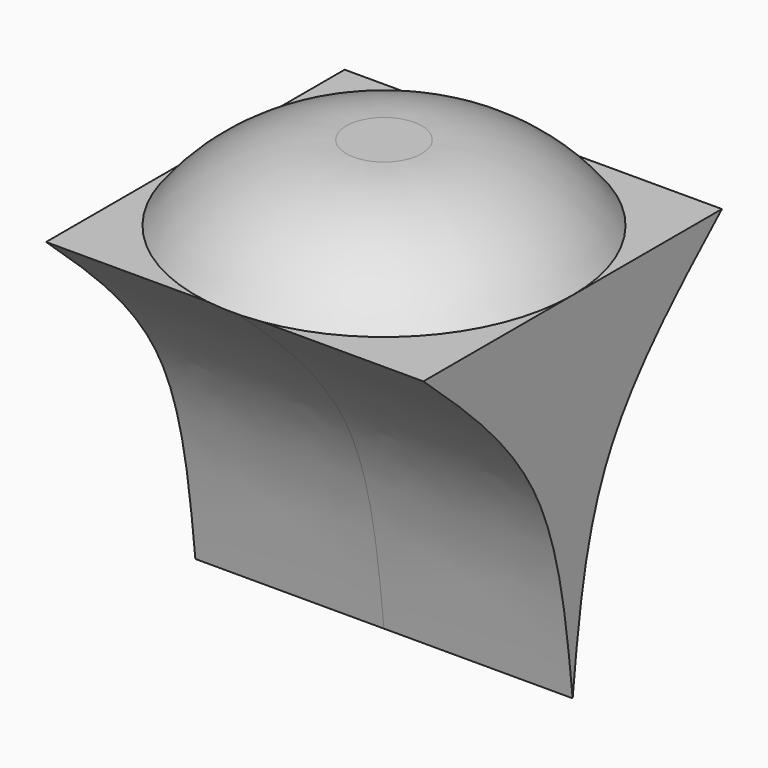
from build123d import *

# Parameters (mm, degrees)
F0_R     = 25
F1_DEPTH = 10
F4_DEPTH = 25
F5_DEPTH = 25


# Not quite as in the source:
# - a fillet or chamfer that OpenCascade refuses, or shapes differently, is made with other operations: its cross-section is extruded or revolved along the edge and cut away or added


with BuildPart() as f1:
    # F0 (on Top) → F1 (new body)
    with BuildSketch(Plane.XY):
        Circle(F0_R)
    extrude(amount=F1_DEPTH)

    # F2: fillet of radius 25 on 1 edges, made by hand

    # F2_s1 → F2_t2 (revolve, cut)
    with BuildSketch(Plane.XZ):
        with BuildLine():
            ThreePointArc((25, 0), (16.1803398875, 7.360679775), (5, 10))
            Line((5, 10), (25, 10))
            Line((25, 10), (25, 0))
        make_face()
    revolve(axis=Axis((0, 0, 10), (0, 0, 1)), mode=Mode.SUBTRACT)

    # F3 (on Right) → F4 (join)
    with BuildSketch(Plane.YZ):
        with BuildLine():
            add(Edge.make_bspline(
                [(24.730604142, 0), (17.4811016216, -6.4583238577), (3.1217539474, -19.2505557941), (1.033815633, -37.8348617707), (0, -47.0366403461)],
                knots=[0, 0, 0, 0, 0.5048629426, 1, 1, 1, 1], degree=3))
            Line((24.730604142, 0), (-24.730604142, 0))
            add(Edge.make_bspline(
                [(-24.730604142, 0), (-17.4811016216, -6.4583238577), (-3.1217539474, -19.2505557941), (-1.033815633, -37.8348617707), (0, -47.0366403461)],
                knots=[0, 0, 0, 0, 0.5048629426, 1, 1, 1, 1], degree=3))
        make_face()
    extrude(amount=F4_DEPTH)

    # F5 (add): a face of the model
    f5_faces = [f1.faces().sort_by_distance(p)[0] for p in [
        (0, 0, -11.4252371801),
    ]]
    extrude(f5_faces, amount=F5_DEPTH)


solid = f1.part
